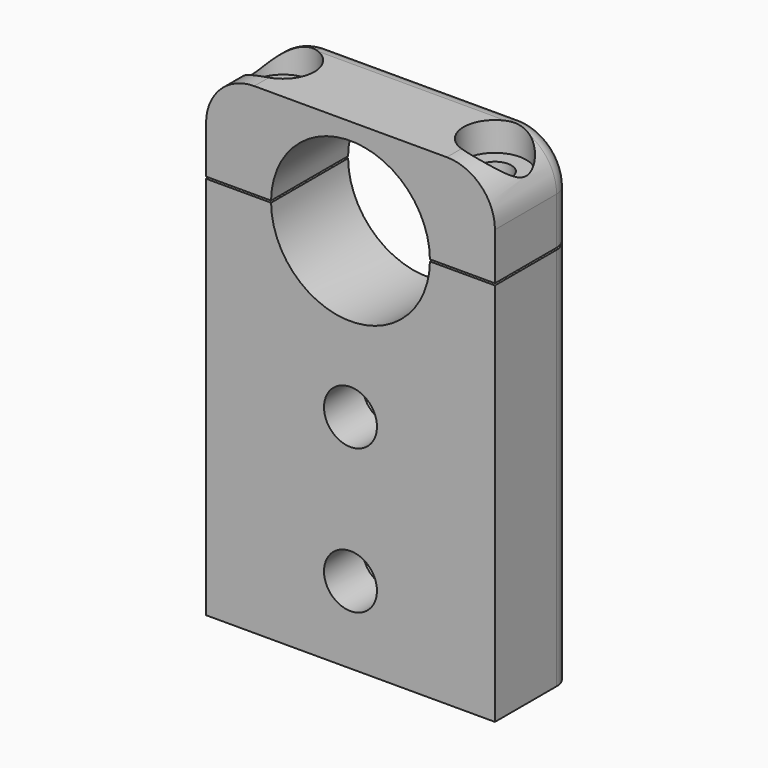
from build123d import *

# Parameters (mm, degrees)
F0_W           = 30
F0_H           = 50
F0_R           = 8.25
F1_DEPTH       = 10
F2_D           = 5.5
F2_CBORE_D     = 9.75
F2_CBORE_DEPTH = 5
F4_D           = 3.4
F4_CBORE_D     = 6.5
F4_CBORE_DEPTH = 3
F5_T1_DEPTH    = 35
F6_R           = 1.7
F7_DEPTH       = 25
F8_T1_DEPTH    = 50
F8_T3_DEPTH    = 20
F8_T6_ANGLE    = 89.9999999974
F8_T8_ANGLE    = 89.9999999974
F9_W           = 50
F9_H           = 0.2
F10_DEPTH      = 25


# Not quite as in the source:
# - a fillet or chamfer that OpenCascade refuses, or shapes differently, is made with other operations: its cross-section is extruded or revolved along the edge and cut away or added


with BuildPart() as f1:
    # F0 (on Front) → F1 (new body)
    with BuildSketch(Plane.XZ):
        with Locations((0, -15)):
            Rectangle(F0_W, F0_H)
        Circle(F0_R, mode=Mode.SUBTRACT)
    extrude(amount=F1_DEPTH)

    # F2 (through all)
    with Locations(Plane(origin=(0, 0, 0), x_dir=(1, 0, 0), z_dir=(0, 1, 0))):
        with Locations((0, 17), (0, 32)):
            CounterBoreHole(F2_D / 2, F2_CBORE_D / 2, F2_CBORE_DEPTH)

    # F4 (through all)
    with Locations(Plane.XY.offset(10)):
        with Locations((11, -5), (-11, -5)):
            CounterBoreHole(F4_D / 2, F4_CBORE_D / 2, F4_CBORE_DEPTH)

    # F5: fillet of radius 5 on 2 edges, made by hand

    # F5_s2 → F5_t1 (cut)
    with BuildSketch(Plane.XZ.offset(-12.5)):
        with BuildLine():
            ThreePointArc((10, 10), (13.5355339059, 8.5355339059), (15, 5))
            Line((15, 5), (15, 10))
            Line((15, 10), (10, 10))
        make_face()
        with BuildLine():
            ThreePointArc((-10, 10), (-13.5355339059, 8.5355339059), (-15, 5))
            Line((-15, 5), (-15, 10))
            Line((-15, 10), (-10, 10))
        make_face()
    extrude(amount=F5_T1_DEPTH, mode=Mode.SUBTRACT)

    # F6 (on face) → F7 (cut)
    with BuildSketch(Plane(origin=(0, 0, -40), x_dir=(1, 0, 0), z_dir=(0, 0, -1))):
        Polygon((11, 8.4641016151), (8, 6.7320508076), (8, 3.2679491924), (11, 1.5358983849), (14, 3.2679491924), (14, 6.7320508076), align=None)
        with Locations((11, 5)):
            Circle(F6_R, mode=Mode.SUBTRACT)
        Polygon((-8, 6.7320508076), (-11, 8.4641016151), (-14, 6.7320508076), (-14, 3.2679491924), (-11, 1.5358983849), (-8, 3.2679491924), align=None)
        with Locations((-11, 5)):
            Circle(F6_R, mode=Mode.SUBTRACT)
    extrude(amount=-F7_DEPTH, mode=Mode.SUBTRACT)

    # F8: fillet of radius 2 on 5 edges, made by hand

    # F8_s2 → F8_t1 (cut)
    with BuildSketch(Plane.XY.offset(-45)):
        with BuildLine():
            ThreePointArc((13, 0), (14.4142135624, -0.5857864376), (15, -2))
            Line((15, -2), (15, 0))
            Line((15, 0), (13, 0))
        make_face()
        with BuildLine():
            ThreePointArc((-13, 0), (-14.4142135624, -0.5857864376), (-15, -2))
            Line((-15, -2), (-15, 0))
            Line((-15, 0), (-13, 0))
        make_face()
    extrude(amount=F8_T1_DEPTH, mode=Mode.SUBTRACT)

    # F8_s4 → F8_t3 (cut)
    with BuildSketch(Plane.YZ.offset(-10)):
        with BuildLine():
            ThreePointArc((-2, 10), (-0.5857864376, 9.4142135624), (0, 8))
            Line((0, 8), (0, 10))
            Line((0, 10), (-2, 10))
        make_face()
    extrude(amount=F8_T3_DEPTH, mode=Mode.SUBTRACT)

    # F8_s5 → F8_t6 (revolve, cut)
    with BuildSketch(Plane.YZ.offset(9.9999999999)):
        with BuildLine():
            ThreePointArc((0, 8), (-0.5857864376, 9.4142135624), (-2, 10))
            Line((-2, 10), (0, 10))
            Line((0, 10), (0, 8))
        make_face()
    revolve(axis=Axis((9.9999999999, 0, 4.9999999999), (0, 1, 0)), revolution_arc=F8_T6_ANGLE, mode=Mode.SUBTRACT)

    # F8_s7 → F8_t8 (revolve, cut)
    with BuildSketch(Plane.XY.offset(4.9999999999)):
        with BuildLine():
            ThreePointArc((-13, 0), (-14.4142135624, -0.5857864376), (-15, -2))
            Line((-15, -2), (-15, 0))
            Line((-15, 0), (-13, 0))
        make_face()
    revolve(axis=Axis((-9.9999999999, 0, 4.9999999999), (0, 1, 0)), revolution_arc=F8_T8_ANGLE, mode=Mode.SUBTRACT)

    # F9 (on face) → F10 (cut)
    with BuildSketch(Plane.XZ):
        Rectangle(F9_W, F9_H)
    extrude(amount=F10_DEPTH, mode=Mode.SUBTRACT)


solid = f1.part
